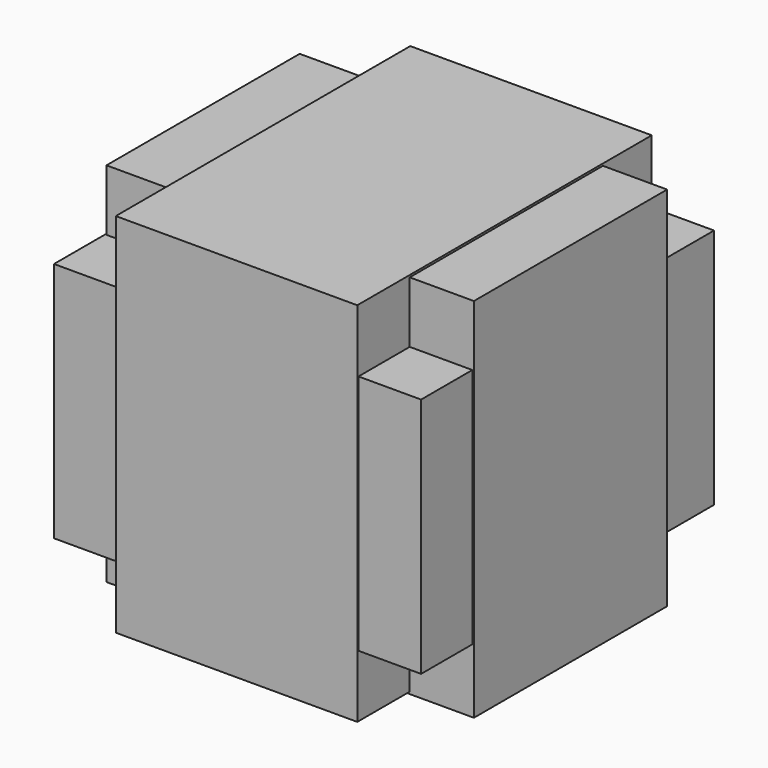
from build123d import *

# Parameters (mm, degrees)
F1_W          = 152.0064324141
F1_H          = 151.6206115484
F3_DEPTH      = 50
F3_DEPTH_BACK = 50
F0_W          = 152.1505489945
F0_H          = 151.9152671099
F4_DEPTH      = 50
F4_DEPTH_BACK = 50
F2_W          = 152.4115279317
F2_H          = 151.8903151155
F5_DEPTH      = 50
F5_DEPTH_BACK = 50


# Not quite as in the source:
# - the program builds the solid bodies; features that only make, move or delete a surface that nothing else refers to are left out


with BuildPart() as f3:
    # F1 (on Top) → F3 (new body, two sides)
    with BuildSketch(Plane.XY) as f3_sk:
        with Locations((-0.0777542591, -0.7124021649)):
            Rectangle(F1_W, F1_H)
    extrude(amount=F3_DEPTH)
    extrude(f3_sk.sketch, amount=-F3_DEPTH_BACK)

    # F0 (on Front) → F4 (join, two sides)
    with BuildSketch(Plane.XZ) as f4_sk:
        with Locations((0.5021430552, -0.6082579494)):
            Rectangle(F0_W, F0_H)
    extrude(amount=F4_DEPTH)
    extrude(f4_sk.sketch, amount=-F4_DEPTH_BACK)

    # F2 (on Right) → F5 (join, two sides)
    with BuildSketch(Plane.YZ) as f5_sk:
        with Locations((-0.9317584336, 0.2604238689)):
            Rectangle(F2_W, F2_H)
    extrude(amount=F5_DEPTH)
    extrude(f5_sk.sketch, amount=-F5_DEPTH_BACK)


solid = f3.part
